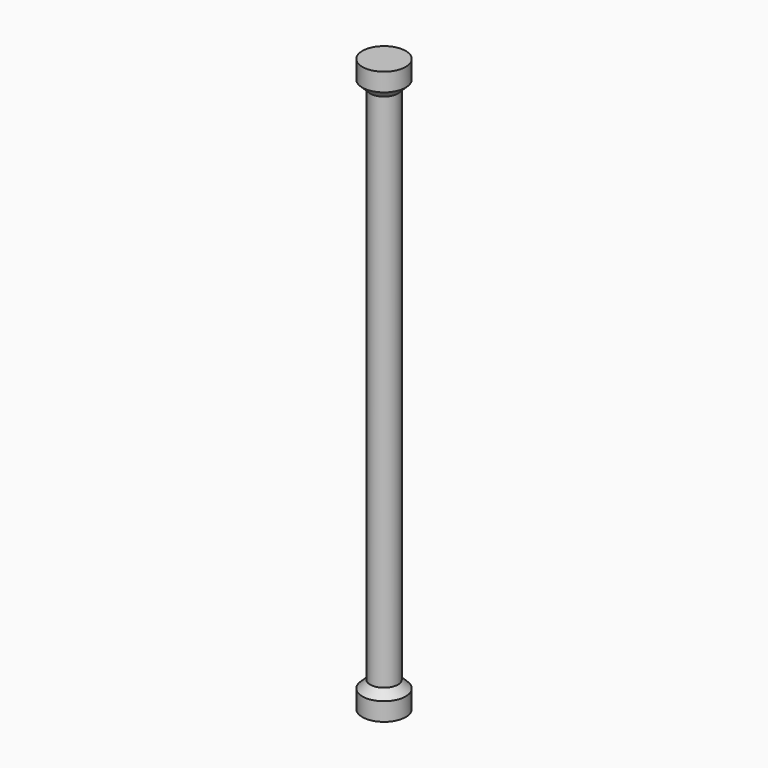
from build123d import *

# Parameters (mm, degrees)
F0_R     = 4.064
F1_DEPTH = 152.4
F2_R     = 6.35
F2_R_2   = 4.064
F3_DEPTH = 7.62
F4_R     = 6.35
F4_R_2   = 4.064
F5_DEPTH = 7.62
F6_SIZE  = 2.28599


# Not quite as in the source:
# - a fillet or chamfer is up to 0.001 mm smaller than in the source, because OpenCascade refuses the exact size


with BuildPart() as f1:
    # F0 (on Top) → F1 (new body)
    with BuildSketch(Plane.XY):
        Circle(F0_R)
    extrude(amount=F1_DEPTH)

    # F2 (on face) → F3 (join)
    with BuildSketch(Plane.XY.offset(152.4)):
        Circle(F2_R)
        Circle(F2_R_2, mode=Mode.SUBTRACT)
        Circle(F2_R_2)
    extrude(amount=F3_DEPTH)

    # F4 (on face) → F5 (join)
    with BuildSketch(Plane(origin=(0, 0, 0), x_dir=(1, 0, 0), z_dir=(0, 0, -1))):
        Circle(F4_R)
        Circle(F4_R_2, mode=Mode.SUBTRACT)
        Circle(F4_R_2)
    extrude(amount=F5_DEPTH)

    # F6 (size 2.286 in the source; OpenCascade refuses exactly that, so slightly less here)
    f6_edges = [f1.edges().sort_by_distance(p)[0] for p in [
        (-6.35, 0, 0),
        (-6.35, 0, 152.4),
    ]]
    chamfer(f6_edges, length=F6_SIZE)


solid = f1.part
